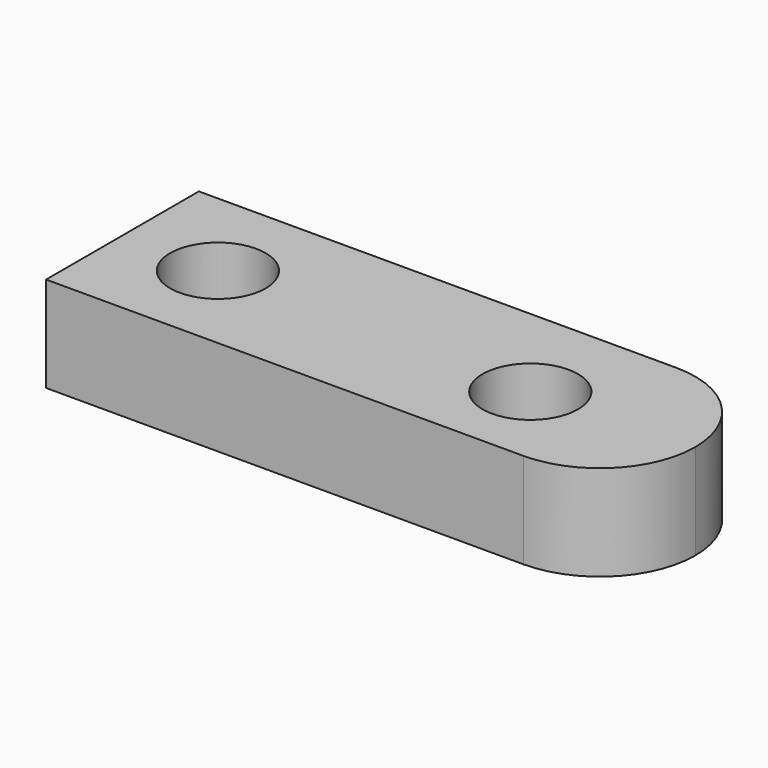
from build123d import *

# Parameters (mm, degrees)
F0_W     = 114.3
F0_H     = 19.05
F1_DEPTH = 38.1
F2_R     = 19.04999
F3_R     = 9.525
F4_DEPTH = 38.1


# Not quite as in the source:
# - a fillet or chamfer is up to 0.001 mm smaller than in the source, because OpenCascade refuses the exact size


with BuildPart() as f1:
    # F0 (on Front) → F1 (new body)
    with BuildSketch(Plane.XZ):
        with Locations((-4.4788396761, 9.525)):
            Rectangle(F0_W, F0_H)
    extrude(amount=F1_DEPTH)

    # F2 (radius 19.05 in the source; OpenCascade refuses exactly that, so slightly less here)
    f2_edges = [f1.edges().sort_by_distance(p)[0] for p in [
        (52.67116, -38.1, 9.525),
        (52.67116, 0, 9.525),
    ]]
    fillet(f2_edges, radius=F2_R)

    # F3 (on face) → F4 (cut)
    with BuildSketch(Plane.XY.offset(19.05)):
        with Locations((-42.5788396761, -19.05)):
            Circle(F3_R)
        with Locations((20.9211603239, -20.5131974071)):
            Circle(F3_R)
    extrude(amount=-F4_DEPTH, mode=Mode.SUBTRACT)


solid = f1.part
